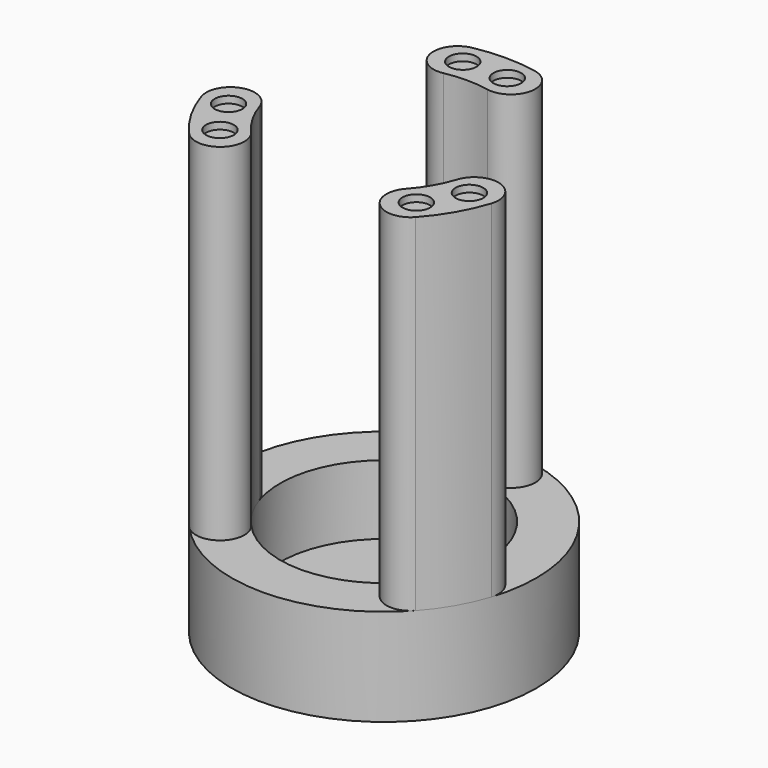
from build123d import *

# Parameters (mm, degrees)
F0_R     = 11
F1_DEPTH = 2
F2_R     = 11
F2_R_2   = 7.5
F3_DEPTH = 5
F5_DEPTH = 25
F6_R     = 1
F7_DEPTH = 0.5


# Not quite as in the source:
# - after a boolean that leaves OpenCascade's solid faulty, fix() repairs it


with BuildPart() as f1:
    # F0 (on Top) → F1 (new body)
    with BuildSketch(Plane.XY):
        Circle(F0_R)
    extrude(amount=F1_DEPTH)

    # F2 (on face) → F3 (join)
    with BuildSketch(Plane.XY.offset(2)):
        Circle(F2_R)
        Circle(F2_R_2, mode=Mode.SUBTRACT)
    extrude(amount=F3_DEPTH)

    # F4 (on face) → F5 (join)
    with BuildSketch(Plane.XY.offset(7)):
        with BuildLine():
            ThreePointArc((1.5866260906, 7.3305332619), (3.640515185, 8.7113082573), (2.2597401896, 10.7651973517))
            ThreePointArc((2.2597401896, 10.7651973517), (0, 10.984539336), (-2.2597401896, 10.7651973517))
            ThreePointArc((-2.2597401896, 10.7651973517), (-3.640515185, 8.7113082573), (-1.5866260906, 7.3305332619))
            ThreePointArc((-1.5866260906, 7.3305332619), (0, 7.484539336), (1.5866260906, 7.3305332619))
        make_face()
        with BuildLine():
            ThreePointArc((5.5735861911, -5.0184795477), (5.7031110745, -7.4899615534), (8.1745930803, -7.3604366699))
            ThreePointArc((8.1745930803, -7.3604366699), (9.5262794416, -5.5), (10.4616216792, -3.3991869381))
            ThreePointArc((10.4616216792, -3.3991869381), (9.3380525159, -1.1940582945), (7.1329238722, -2.3176274578))
            ThreePointArc((7.1329238722, -2.3176274578), (6.4951905284, -3.75), (5.5735861911, -5.0184795477))
        make_face()
        with BuildLine():
            ThreePointArc((-7.1329238722, -2.3176274578), (-9.3380525159, -1.1940582945), (-10.4616216792, -3.3991869381))
            ThreePointArc((-10.4616216792, -3.3991869381), (-9.5262794416, -5.5), (-8.1745930803, -7.3604366699))
            ThreePointArc((-8.1745930803, -7.3604366699), (-5.7031110745, -7.4899615534), (-5.5735861911, -5.0184795477))
            ThreePointArc((-5.5735861911, -5.0184795477), (-6.4951905284, -3.75), (-7.1329238722, -2.3176274578))
        make_face()
    extrude(amount=F5_DEPTH)

    add(f1.part.fix(), mode=Mode.REPLACE)

    # F6 (on face) → F7 (cut)
    with BuildSketch(Plane.XY.offset(32)):
        with Locations((-1.6062456434, 9.1094717154)):
            Circle(F6_R)
        with Locations((-7.0859110989, -5.9457853896)):
            Circle(F6_R)
        with Locations((1.6062456434, 9.1094717154)):
            Circle(F6_R)
        with Locations((-8.6921567423, -3.1636863258)):
            Circle(F6_R)
        with Locations((8.6921567423, -3.1636863258)):
            Circle(F6_R)
        with Locations((7.0859110989, -5.9457853896)):
            Circle(F6_R)
    extrude(amount=-F7_DEPTH, mode=Mode.SUBTRACT)


solid = f1.part
